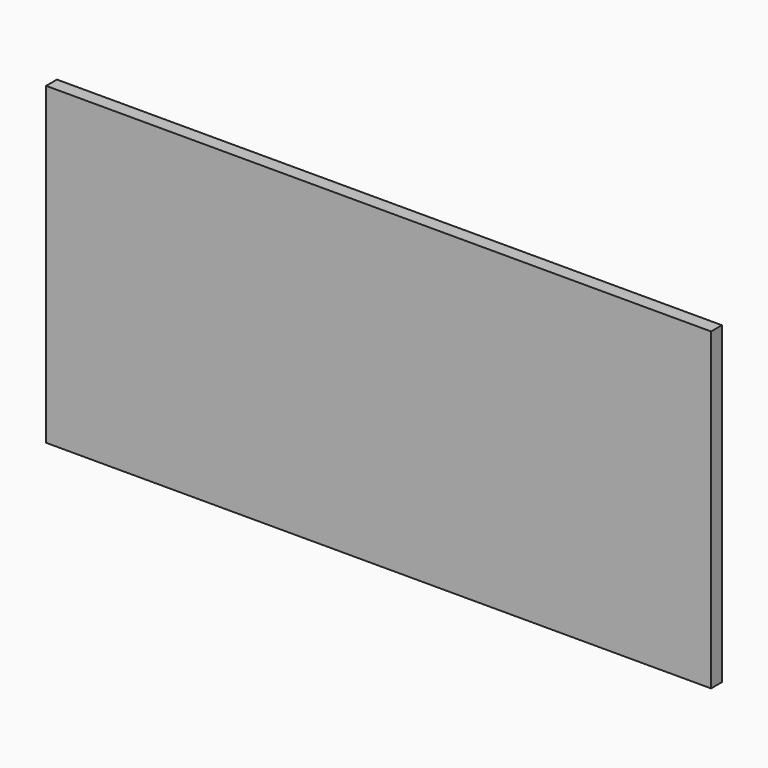
from build123d import *

# Parameters (mm, degrees)
F0_W     = 603.25
F0_H     = 279.4
F2_DEPTH = 12.065
F3_DEPTH = 6.0325
F4_DEPTH = 6.0325


# Not quite as in the source:
# - a variable given as a bare number and used for a length is read in inches; the dataset says mm whatever the document's units were


with BuildPart() as f2:
    # F0 (on Front) → F2 (new body)
    with BuildSketch(Plane.XZ):
        Rectangle(F0_W, F0_H)
    extrude(amount=F2_DEPTH)

    # F3 (cut): a face of the model
    f3_faces = [f2.faces().sort_by_distance(p)[0] for p in [
        (301.625, -6.0325, 0),
    ]]
    extrude(f3_faces, amount=-F3_DEPTH, mode=Mode.SUBTRACT)

    # F4 (cut): a face of the model
    f4_faces = [f2.faces().sort_by_distance(p)[0] for p in [
        (-301.625, -6.0325, 0),
    ]]
    extrude(f4_faces, amount=-F4_DEPTH, mode=Mode.SUBTRACT)


solid = f2.part
